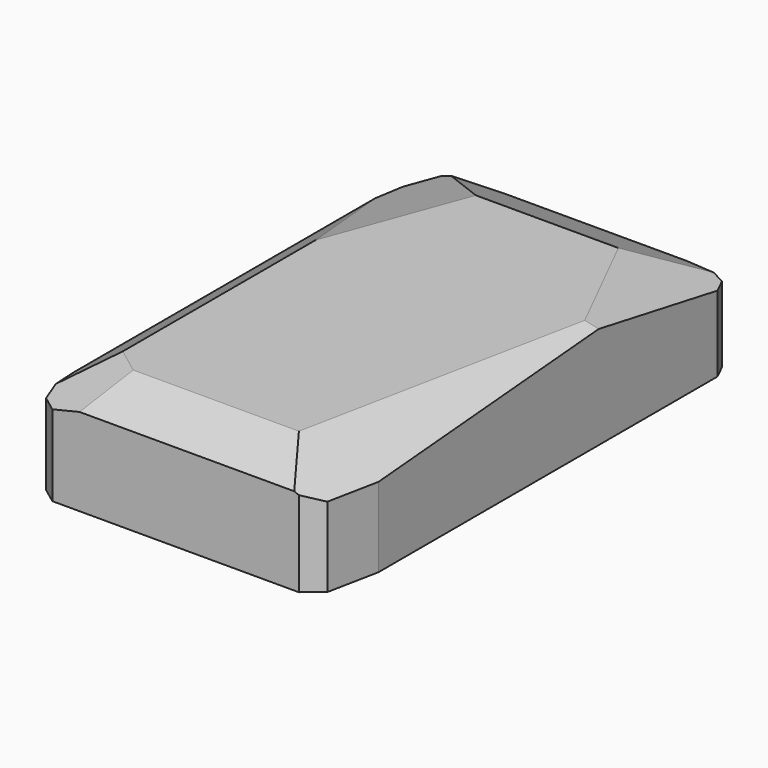
from build123d import *

# Parameters (mm, degrees)
F0_W          = 35.2
F0_H          = 68.2
F1_DEPTH      = 10
F2_W          = 6.5
F2_H          = 14
F3_DEPTH      = 0.5
F4_W          = 37.2
F4_H          = 70.2
F5_DEPTH      = 1.2
F6_W          = 46
F6_H          = 79
F6_W_2        = 41.2
F6_H_2        = 74.2
F7_DEPTH      = 11.2
F7_DEPTH_BACK = 0.2
F8_W          = 46
F8_H          = 79
F9_DEPTH      = 5
F10_T1_DEPTH  = 68.3626417259
F11_SIZE2     = 4
F11_SIZE      = 3
F12_T1_DEPTH  = 51.679588215
F13_T1_DEPTH  = 37.1186309903
F14_T1_DEPTH  = 105.3432147832
F15_T1_DEPTH  = 56.8622727826
F16_T1_DEPTH  = 113.8975360582
F17_T1_DEPTH  = 66.7068632941
F18_T1_DEPTH  = 64.9639966922
F19_T1_DEPTH  = 78.1392222347
F20_SIZE2     = 3
F20_SIZE      = 8
F21_SIZE      = 2.2
F22_SIZE2     = 2
F22_SIZE      = 8
F23_SIZE2     = 2
F23_SIZE      = 6
F24_SIZE2     = 2
F24_SIZE      = 6


# Not quite as in the source:
# - a fillet or chamfer that OpenCascade refuses, or shapes differently, is made with other operations: its cross-section is extruded or revolved along the edge and cut away or added


with BuildPart() as f1:
    # F0 (on Top) → F1 (new body)
    with BuildSketch(Plane.XY):
        Rectangle(F0_W, F0_H)
    extrude(amount=F1_DEPTH)

    # F2 (on face) → F3 (cut)
    with BuildSketch(Plane.XY.offset(10)):
        with Locations((13.35, -26)):
            Rectangle(F2_W, F2_H)
    extrude(amount=-F3_DEPTH, mode=Mode.SUBTRACT)


with BuildPart() as f5:
    # F4 (on face) → F5 (new body)
    with BuildSketch(Plane(origin=(0, 0, 0), x_dir=(1, 0, 0), z_dir=(0, 0, -1))):
        Rectangle(F4_W, F4_H)
    extrude(amount=F5_DEPTH)


with BuildPart() as f7:
    # F6 (on face) → F7 (new body, two sides)
    with BuildSketch(Plane.XY.offset(10)) as f7_sk:
        Rectangle(F6_W, F6_H)
        Rectangle(F6_W_2, F6_H_2, mode=Mode.SUBTRACT)
    extrude(amount=-F7_DEPTH)
    extrude(f7_sk.sketch, amount=F7_DEPTH_BACK)

    # F8 (on face) → F9 (join)
    with BuildSketch(Plane.XY.offset(10.2)):
        Rectangle(F8_W, F8_H)
    extrude(amount=F9_DEPTH)

    # F10: chamfer of 2 x 10 on 1 edges, made by hand

    # F10_s2 → F10_t1 (cut)
    with BuildSketch(Plane.XY.offset(-27.181320863)):
        Polygon((23, -29.5), (21, -39.5), (23, -39.5), align=None)
    extrude(amount=F10_T1_DEPTH, mode=Mode.SUBTRACT)

    # F11
    f11_edges = [f7.edges().sort_by_distance(p)[0] for p in [
        (-23, -39.5, 7),
    ]]
    chamfer(f11_edges, length=F11_SIZE, length2=F11_SIZE2)

    # F12: chamfer of 2.5 x 6.8 on 1 edges, made by hand

    # F12_s2 → F12_t1 (cut)
    with BuildSketch(Plane.XY.offset(-18.8397941075)):
        Polygon((-23, 32.7), (-20.5, 39.5), (-23, 39.5), align=None)
    extrude(amount=F12_T1_DEPTH, mode=Mode.SUBTRACT)

    # F13: chamfer of 4 x 2 on 1 edges, made by hand

    # F13_s2 → F13_t1 (cut)
    with BuildSketch(Plane.XY.offset(-11.5593154951)):
        Polygon((21, 39.5), (23, 35.5), (23, 39.5), align=None)
    extrude(amount=F13_T1_DEPTH, mode=Mode.SUBTRACT)

    # F14: chamfer of 14 x 4.6 on 1 edges, made by hand

    # F14_s2 → F14_t1 (cut)
    with BuildSketch(Plane(origin=(22.8891289585, 62.258430767, 0), x_dir=(0, 0, 1), z_dir=(-0.3450656446, -0.9385785534, 0))):
        Polygon((10.6, 32.8709533075), (15.2, 18.8709533075), (15.2, 32.8709533075), align=None)
    extrude(amount=F14_T1_DEPTH, mode=Mode.SUBTRACT)

    # F15: chamfer of 10 x 4 on 1 edges, made by hand

    # F15_s2 → F15_t1 (cut)
    with BuildSketch(Plane(origin=(-17.944909113, 13.4586818348, 0), x_dir=(0, 0, 1), z_dir=(0.8, -0.6, 0))):
        Polygon((11.2, 43), (15.2, 33), (15.2, 43), align=None)
    extrude(amount=F15_T1_DEPTH, mode=Mode.SUBTRACT)

    # F16: chamfer of 10 x 4.2 on 1 edges, made by hand

    # F16_s2 → F16_t1 (cut)
    with BuildSketch(Plane(origin=(-11.8727476818, -59.3637384092, 0), x_dir=(0, 0, 1), z_dir=(0.1961161351, 0.9805806757, 0))):
        Polygon((11, 28.3387815275), (15.2, 18.3387815275), (15.2, 28.3387815275), align=None)
    extrude(amount=F16_T1_DEPTH, mode=Mode.SUBTRACT)

    # F17: chamfer of 12 x 4.8 on 1 edges, made by hand

    # F17_s2 → F17_t1 (cut)
    with BuildSketch(Plane(origin=(4.3161080891, -8.6322161783, 0), x_dir=(0, 0, 1), z_dir=(-0.4472135955, 0.894427191, 0))):
        Polygon((10.4, 36.4479080332), (15.2, 24.4479080332), (15.2, 36.4479080332), align=None)
    extrude(amount=F17_T1_DEPTH, mode=Mode.SUBTRACT)

    # F18: chamfer of 5 x 10 on 1 edges, made by hand

    # F18_s2 → F18_t1 (cut)
    with BuildSketch(Plane.YZ.offset(-31.4821158194)):
        Polygon((39.5, 10.2), (29.5, 15.2), (39.5, 15.2), align=None)
    extrude(amount=F18_T1_DEPTH, mode=Mode.SUBTRACT)

    # F19: chamfer of 4 x 6 on 1 edges, made by hand

    # F19_s2 → F19_t1 (cut)
    with BuildSketch(Plane.XZ.offset(-38.6364190914)):
        Polygon((-23, 11.2), (-17, 15.2), (-23, 15.2), align=None)
    extrude(amount=F19_T1_DEPTH, mode=Mode.SUBTRACT)

    # F20
    f20_edges = [f7.edges().sort_by_distance(p)[0] for p in [
        (4.234314, -39.5, 15.2),
    ]]
    f20_side = f7.faces().sort_by_distance((0.719932, -3.706312, 15.2))[0]
    chamfer(f20_edges, length=F20_SIZE, length2=F20_SIZE2, reference=f20_side)

    # F21
    f21_edges = [f7.edges().sort_by_distance(p)[0] for p in [
        (21, -39.5, 4.9),
    ]]
    chamfer(f21_edges, length=F21_SIZE)

    # F22
    f22_edges = [f7.edges().sort_by_distance(p)[0] for p in [
        (-20.5, 39.5, 4.5),
    ]]
    chamfer(f22_edges, length=F22_SIZE, length2=F22_SIZE2)

    # F23
    f23_edges = [f7.edges().sort_by_distance(p)[0] for p in [
        (21, 39.5, 4.5),
    ]]
    chamfer(f23_edges, length=F23_SIZE, length2=F23_SIZE2)

    # F24
    f24_edges = [f7.edges().sort_by_distance(p)[0] for p in [
        (-23, -36.5, 5),
    ]]
    chamfer(f24_edges, length=F24_SIZE, length2=F24_SIZE2)


solid = Compound([f1.part, f5.part, f7.part])
